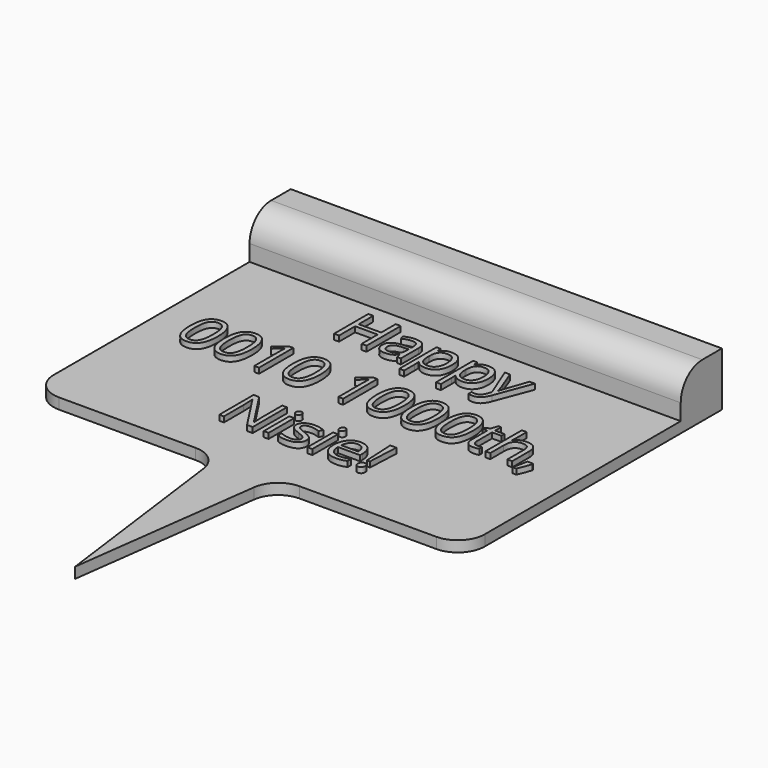
from build123d import *

# Parameters (mm, degrees)
F1_DEPTH     = 2
F2_TEXT_SIZE = 11.1111111111
F3_DEPTH     = 1
F4_W         = 80
F4_H         = 9.5521336794
F5_DEPTH     = 8
F6_R         = 3
F7_DEPTH     = 8
F8_R         = 5


# Not quite as in the source:
# - Text() gives the source's letters only with a copy of the font that has no kerning and outlines rounded to 1/6400 em; it was checked with that copy


with BuildPart() as f1:
    # F0 (on Top) → F1 (new body)
    with BuildSketch(Plane.XY):
        Polygon((-40, 60), (-40, 0), (-5.2660999035, 0), (5.2660999035, 0), (40, 0), (40, 60), align=None)
        Polygon((5.2660999035, 0), (-5.2660999035, 0), (0, -40), align=None)
    extrude(amount=F1_DEPTH)

    # F2 (on face) → F3 (join)
    with BuildSketch(Plane.XY.offset(2)):
        with Locations((-16.2517361111, 39)):
            Text('Happy', F2_TEXT_SIZE, font='Open Sans', text_align=(TextAlign.LEFT, TextAlign.BOTTOM))
        with Locations((-33.5746527778, 23.8888888889)):
            Text('0010 1000th,', F2_TEXT_SIZE, font='Open Sans', text_align=(TextAlign.LEFT, TextAlign.BOTTOM))
        with Locations((-13.3645833333, 8.7777777778)):
            Text('Nisie!', F2_TEXT_SIZE, font='Open Sans', text_align=(TextAlign.LEFT, TextAlign.BOTTOM))
    extrude(amount=F3_DEPTH)

    # F4 (on face) → F5 (join)
    with BuildSketch(Plane.XY.offset(2)):
        with Locations((0, 55.2239331603)):
            Rectangle(F4_W, F4_H)
    extrude(amount=F5_DEPTH)

    # F6 (on face) → F7 (cut)
    with BuildSketch(Plane(origin=(0, 60, 0), x_dir=(-1, 0, 0), z_dir=(0, 1, 0))):
        with Locations((35, 5)):
            Circle(F6_R)
        with Locations((25, 5)):
            Circle(F6_R)
        with Locations((15, 5)):
            Circle(F6_R)
        with Locations((5, 5)):
            Circle(F6_R)
        with Locations((-5, 5)):
            Circle(F6_R)
        with Locations((-15, 5)):
            Circle(F6_R)
        with Locations((-25, 5)):
            Circle(F6_R)
        with Locations((-35, 5)):
            Circle(F6_R)
    extrude(amount=-F7_DEPTH, mode=Mode.SUBTRACT)

    # F8
    f8_edges = [f1.edges().sort_by_distance(p)[0] for p in [
        (0, 50.447866, 10),
        (-40, 0, 1),
        (40, 0, 1),
        (5.2661, 0, 1),
        (-5.2661, 0, 1),
    ]]
    fillet(f8_edges, radius=F8_R)


solid = f1.part
